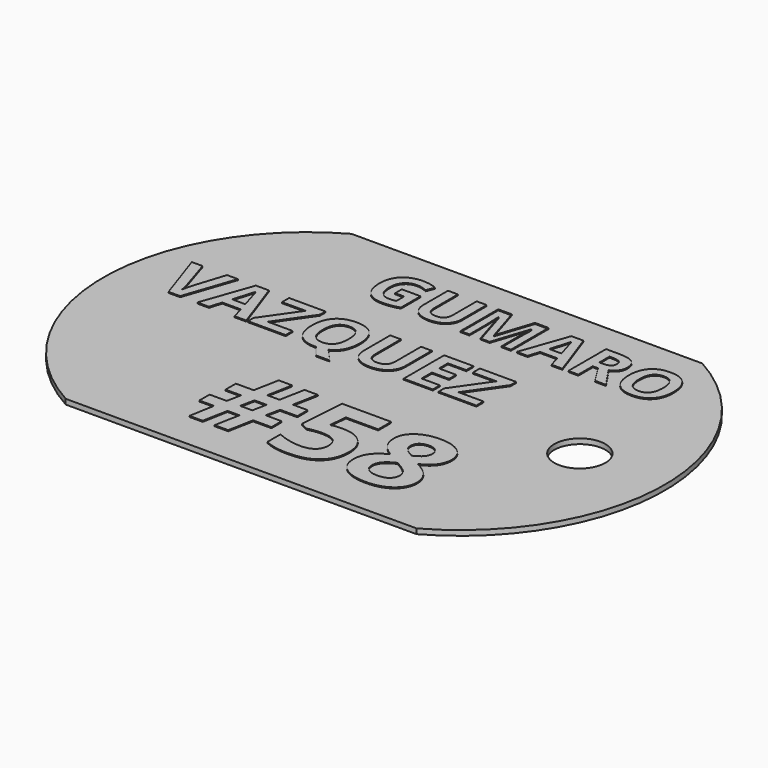
from build123d import *

# Parameters (mm, degrees)
F1_DEPTH       = 0.635
F3_D           = 6.35
F4_TEXT_SIZE   = 8.2169892266
F4_TEXT_SIZE_2 = 8.8194444444
F4_TEXT_SIZE_3 = 15.7707849414
F5_DEPTH       = 0.127
F6_TEXT_SIZE   = 33.0675483888
F6_TEXT_SIZE_2 = 33.0675496823
F7_DEPTH       = 0.127


# Not quite as in the source:
# - Text() gives the source's letters only with a copy of the font that has no kerning and outlines rounded to 1/6400 em; it was checked with that copy


with BuildPart() as f1:
    # F0 (on Top) → F1 (new body)
    with BuildSketch(Plane.XY):
        with BuildLine():
            Line((-21.8217221242, -22.225), (21.8217221242, -22.225))
            ThreePointArc((21.8217221242, -22.225), (34.925, 0), (21.8217221242, 22.225))
            Line((21.8217221242, 22.225), (-21.8217221242, 22.225))
            ThreePointArc((-21.8217221242, 22.225), (-34.925, 0), (-21.8217221242, -22.225))
        make_face()
    extrude(amount=F1_DEPTH)

    # F3 (through all)
    with Locations(Plane.XY.offset(0.635)):
        with Locations((24.3695825338, 0)):
            Hole(F3_D / 2)

    # F4 (on face) → F5 (join)
    with BuildSketch(Plane.XY.offset(0.635)):
        with Locations((-13.5228177533, 12.6776434481)):
            Text('GUMARO', F4_TEXT_SIZE, font='Open Sans', font_style=FontStyle.BOLD, text_align=(TextAlign.LEFT, TextAlign.BOTTOM))
        with Locations((-30.0798046105, 1.4086279552)):
            Text('VAZQUEZ', F4_TEXT_SIZE_2, font='Open Sans', font_style=FontStyle.BOLD, text_align=(TextAlign.LEFT, TextAlign.BOTTOM))
        with Locations((-11.6591406986, -17.7037958056)):
            Text('#58', F4_TEXT_SIZE_3, font='Open Sans', font_style=FontStyle.BOLD, text_align=(TextAlign.LEFT, TextAlign.BOTTOM))
    extrude(amount=F5_DEPTH)

    # F6 (on face) → F7 (join)
    with BuildSketch(Plane(origin=(0, 0, 0), x_dir=(1, 0, 0), z_dir=(0, 0, -1))):
        with Locations((-32.0938080549, -9.8689300939)):
            Text('M', F6_TEXT_SIZE, font='Open Sans', font_style=FontStyle.BOLD, text_align=(TextAlign.LEFT, TextAlign.BOTTOM))
        with Locations((0, -9.8689310253)):
            Text('K', F6_TEXT_SIZE_2, font='Open Sans', text_align=(TextAlign.LEFT, TextAlign.BOTTOM))
    extrude(amount=F7_DEPTH)


solid = f1.part
